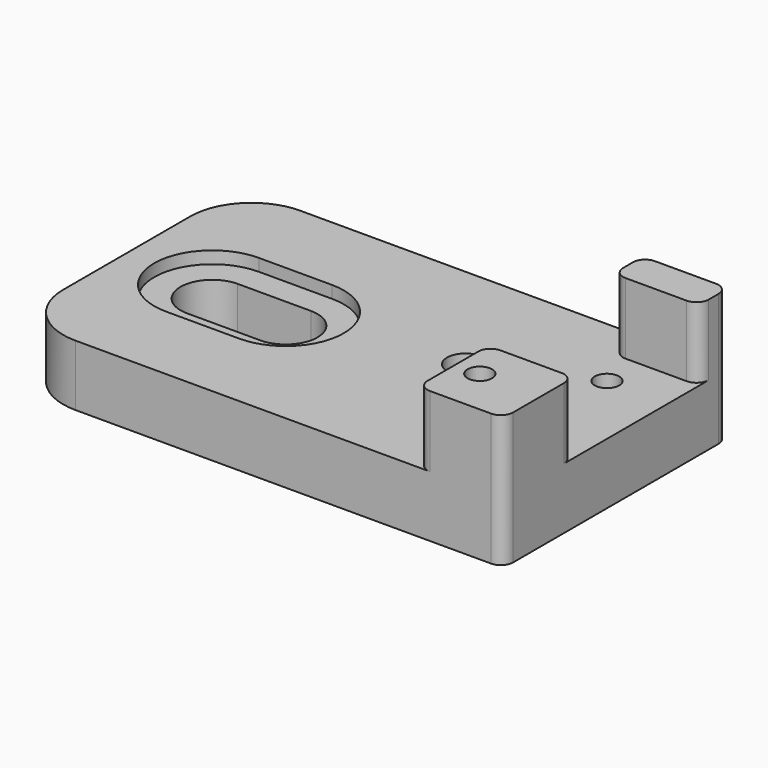
from build123d import *

# Parameters (mm, degrees)
F0_W     = 20
F0_H     = 23
F1_DEPTH = 5
F2_W     = 7
F2_H     = 3
F2_H_2   = 7.2
F2_R     = 1
F3_DEPTH = 5.8
F4_DEPTH = 5.001
F5_R     = 5
F6_R     = 1
F7_R     = 1
F8_DEPTH = 4
F2_R_2   = 1.5
F9_DEPTH = 5.001


with BuildPart() as f1:
    # F0 (on Top) → F1 (new body)
    with BuildSketch(Plane.XY):
        Rectangle(F0_W, F0_H)
        with BuildLine():
            Line((-3, 4.75), (3, 4.75))
            ThreePointArc((3, 4.75), (7.75, 0), (3, -4.75))
            Line((3, -4.75), (-3, -4.75))
            ThreePointArc((-3, -4.75), (-7.75, 0), (-3, 4.75))
        make_face(mode=Mode.SUBTRACT)
        with Locations((20, 0)):
            Rectangle(F0_W, F0_H)
    extrude(amount=F1_DEPTH)

    # F2 (on face) → F3 (join)
    with BuildSketch(Plane.XY.offset(5)):
        with Locations((26.5, 10)):
            Rectangle(F2_W, F2_H)
        with Locations((26.5, -7.9)):
            Rectangle(F2_W, F2_H_2)
        with Locations((25, -7.65)):
            Circle(F2_R, mode=Mode.SUBTRACT)
    extrude(amount=F3_DEPTH)

    # F2 (on face) → F4 (cut, through all)
    with BuildSketch(Plane.XY.offset(5)):
        with Locations((25, 5.35)):
            Circle(F2_R)
        with Locations((25, -1.15)):
            Circle(F2_R)
        with Locations((25, -7.65)):
            Circle(F2_R)
    extrude(amount=-F4_DEPTH, mode=Mode.SUBTRACT)

    # F5
    f5_edges = [f1.edges().sort_by_distance(p)[0] for p in [
        (-10, -11.5, 2.5),
        (-10, 11.5, 2.5),
    ]]
    fillet(f5_edges, radius=F5_R)

    # F6
    f6_edges = [f1.edges().sort_by_distance(p)[0] for p in [
        (30, -11.5, 5.4),
        (30, 11.5, 5.4),
    ]]
    fillet(f6_edges, radius=F6_R)

    # F7
    f7_edges = [f1.edges().sort_by_distance(p)[0] for p in [
        (23, 8.5, 7.9),
        (23, -4.3, 7.9),
        (30, -4.3, 7.9),
        (30, 8.5, 7.9),
        (23, -11.5, 7.9),
        (23, 11.5, 7.9),
    ]]
    fillet(f7_edges, radius=F7_R)

    # F0 (on Top) → F8 (join)
    with BuildSketch(Plane.XY):
        with BuildLine():
            ThreePointArc((3, -4.75), (7.75, 0), (3, 4.75))
            Line((3, 4.75), (-3, 4.75))
            ThreePointArc((-3, 4.75), (-7.75, 0), (-3, -4.75))
            Line((-3, -4.75), (3, -4.75))
        make_face()
        with BuildLine():
            Line((-3, 2.6), (3, 2.6))
            ThreePointArc((3, 2.6), (5.6, 0), (3, -2.6))
            Line((3, -2.6), (-3, -2.6))
            ThreePointArc((-3, -2.6), (-5.6, 0), (-3, 2.6))
        make_face(mode=Mode.SUBTRACT)
    extrude(amount=F8_DEPTH)

    # F2 (on face) → F9 (cut, through all)
    with BuildSketch(Plane.XY.offset(5)):
        with Locations((16.5, 1.5)):
            Circle(F2_R_2)
    extrude(amount=-F9_DEPTH, mode=Mode.SUBTRACT)


solid = f1.part
